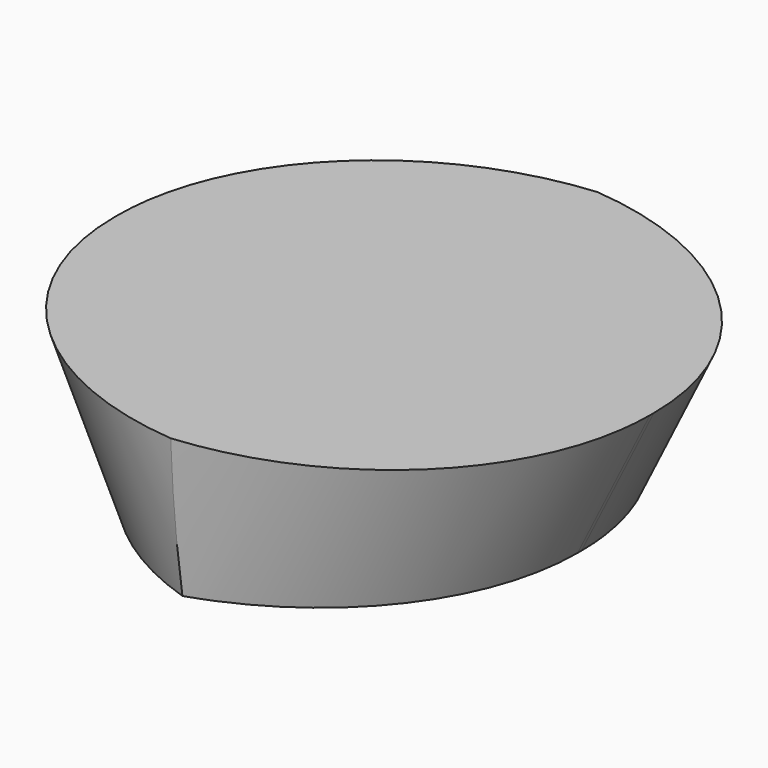
from build123d import *

# Parameters (mm, degrees)
F1_DEPTH    = 1.4097
F2_T1_DEPTH = 7.8369418994
F2_T3_DEPTH = 7.8369418994


# Not quite as in the source:
# - a fillet or chamfer that OpenCascade refuses, or shapes differently, is made with other operations: its cross-section is extruded or revolved along the edge and cut away or added


with BuildPart() as f1:
    # F0 (on Front) → F1 (new body, symmetric)
    with BuildSketch(Plane.XZ):
        Polygon((-1.0287, -0.381), (1.0287, -0.381), (1.4097, 0.381), (-1.4097, 0.381), align=None)
    extrude(amount=F1_DEPTH, both=True)

    # F2: fillet of radius 1.397 on 4 edges, made by hand

    # F2_s2 → F2_t1 (cut)
    with BuildSketch(Plane(origin=(-1.9962334823, 0, 3.9924669646), x_dir=(0, 1, 0), z_dir=(0.4472135955, 0, -0.894427191))):
        with BuildLine():
            ThreePointArc((0.0127, -1.0904856313), (1.0005281733, -0.6813138046), (1.4097, 0.3065143687))
            Line((1.4097, 0.3065143687), (1.4097, -1.0904856313))
            Line((1.4097, -1.0904856313), (0.0127, -1.0904856313))
        make_face()
        with BuildLine():
            ThreePointArc((-0.0127, -1.0904856313), (-1.0005281733, -0.6813138046), (-1.4097, 0.3065143687))
            Line((-1.4097, 0.3065143687), (-1.4097, -1.0904856313))
            Line((-1.4097, -1.0904856313), (-0.0127, -1.0904856313))
        make_face()
    extrude(amount=F2_T1_DEPTH, mode=Mode.SUBTRACT)

    # F2_s4 → F2_t3 (cut)
    with BuildSketch(Plane(origin=(-1.5085534823, 0, -3.0171069646), x_dir=(0, 1, 0), z_dir=(0.4472135955, 0, 0.894427191))):
        with BuildLine():
            ThreePointArc((-1.4097, 0.3065143687), (-1.0005281733, -0.6813138046), (-0.0127, -1.0904856313))
            Line((-0.0127, -1.0904856313), (-1.4097, -1.0904856313))
            Line((-1.4097, -1.0904856313), (-1.4097, 0.3065143687))
        make_face()
        with BuildLine():
            ThreePointArc((0.0127, -1.0904856313), (1.0005281733, -0.6813138046), (1.4097, 0.3065143687))
            Line((1.4097, 0.3065143687), (1.4097, -1.0904856313))
            Line((1.4097, -1.0904856313), (0.0127, -1.0904856313))
        make_face()
    extrude(amount=F2_T3_DEPTH, mode=Mode.SUBTRACT)


solid = f1.part
